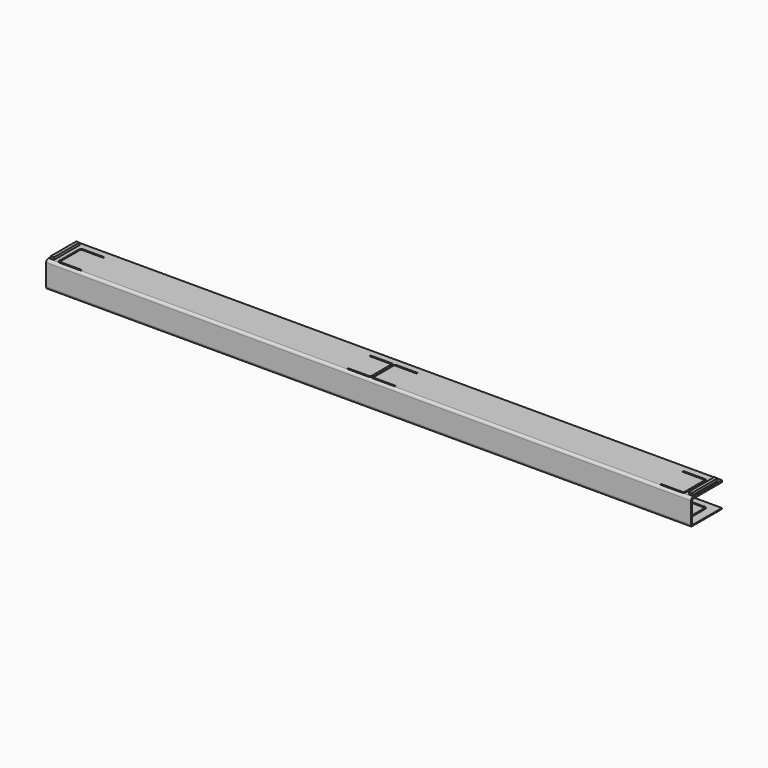
from build123d import *

# Parameters (mm, degrees)
F0_W         = 69
F0_H         = 5.7454954955
F1_DEPTH     = 2050
F2_W         = 10
F2_H         = 101.5
F3_DEPTH     = 7.5
F7_DEPTH     = 84
F10_DEPTH    = 90
F11_T1_DEPTH = 134.5
F12_T1_DEPTH = 139.5


# Not quite as in the source:
# - a fillet or chamfer that OpenCascade refuses, or shapes differently, is made with other operations: its cross-section is extruded or revolved along the edge and cut away or added


with BuildPart() as f1:
    # F0 (on Right) → F1 (new body)
    with BuildSketch(Plane.YZ):
        with BuildLine():
            ThreePointArc((-53.5, -33.75), (-51.1568542495, -39.4068542495), (-45.5, -41.75))
            Line((-45.5, -41.75), (0, -41.75))
            Line((0, -41.75), (0, -36.0045045045))
            Line((0, -36.0045045045), (-45.5, -36.0045045045))
            ThreePointArc((-45.5, -36.0045045045), (-48.3284271247, -34.8329316293), (-49.5, -32.0045045045))
            Line((-49.5, -32.0045045045), (-49.5, 32.0045045045))
            ThreePointArc((-49.5, 32.0045045045), (-48.3284271247, 34.8329316293), (-45.5, 36.0045045045))
            Line((-45.5, 36.0045045045), (0, 36.0045045045))
            Line((0, 36.0045045045), (0, 41.75))
            Line((0, 41.75), (-45.5, 41.75))
            ThreePointArc((-45.5, 41.75), (-51.1568542495, 39.4068542495), (-53.5, 33.75))
            Line((-53.5, 33.75), (-53.5, -33.75))
        make_face()
        with Locations((34.5, 38.8772522523)):
            Rectangle(F0_W, F0_H)
        with Locations((34.5, -38.8772522523)):
            Rectangle(F0_W, F0_H)
    extrude(amount=-F1_DEPTH)

    # F2 (on face) → F3 (join)
    with BuildSketch(Plane.XY.offset(41.75)):
        with Locations((-2039, 8.25)):
            Rectangle(F2_W, F2_H)
    extrude(amount=F3_DEPTH)

    # F5: F1 across plane


with BuildPart() as f1_1:
    add(f1.part)
    add(f1.part.mirror(Plane.YZ.offset(-1025)))

    # F6 (on face) → F7 (cut)
    with BuildSketch(Plane.XY.offset(41.75)):
        with BuildLine():
            Line((-2021, 39.5), (-2021, 0))
            Line((-2021, 0), (-2021, -37.5))
            ThreePointArc((-2021, -37.5), (-2018.6568542495, -43.1568542495), (-2013, -45.5))
            Line((-2013, -45.5), (-1945.5, -45.5))
            Line((-1945.5, -45.5), (-1945.5, -41.25))
            Line((-1945.5, -41.25), (-2004.9698543549, -41.25))
            Line((-2004.9698543549, -41.25), (-2012.75, -41.25))
            ThreePointArc((-2012.75, -41.25), (-2015.5784271247, -40.0784271247), (-2016.75, -37.25))
            Line((-2016.75, -37.25), (-2016.75, 0))
            Line((-2016.75, 0), (-2016.75, 39.25))
            ThreePointArc((-2016.75, 39.25), (-2015.5784271247, 42.0784271247), (-2012.75, 43.25))
            Line((-2012.75, 43.25), (-1945.5, 43.25))
            Line((-1945.5, 43.25), (-1945.5, 47.5))
            Line((-1945.5, 47.5), (-2013, 47.5))
            ThreePointArc((-2013, 47.5), (-2018.6568542495, 45.1568542495), (-2021, 39.5))
        make_face()
    extrude(amount=-F7_DEPTH, mode=Mode.SUBTRACT)

    # F8: F1 across plane


with BuildPart() as f1_2:
    add(f1_1.part)
    add(f1_1.part.mirror(Plane.YZ.offset(-1025)), mode=Mode.INTERSECT)

    # F9 (on face) → F10 (cut)
    with BuildSketch(Plane.XY.offset(41.75)):
        with BuildLine():
            ThreePointArc((-1024.0666470126, -40.75), (-1021.1231056256, -43.8556546004), (-1017, -45))
            Line((-1017, -45), (-950, -45))
            Line((-950, -45), (-950, -40.75))
            Line((-950, -40.75), (-1016.75, -40.75))
            ThreePointArc((-1016.75, -40.75), (-1019.5784271247, -39.5784271247), (-1020.75, -36.75))
            Line((-1020.75, -36.75), (-1020.75, 1.25))
            Line((-1020.75, 1.25), (-1020.75, 39.25))
            ThreePointArc((-1020.75, 39.25), (-1019.5784271247, 42.0784271247), (-1016.75, 43.25))
            Line((-1016.75, 43.25), (-950, 43.25))
            Line((-950, 43.25), (-950, 47.5))
            Line((-950, 47.5), (-1017, 47.5))
            ThreePointArc((-1017, 47.5), (-1021.1231056256, 46.3556546004), (-1024.0666470126, 43.25))
            Line((-1024.0666470126, 43.25), (-1025.9333529874, 43.25))
            ThreePointArc((-1025.9333529874, 43.25), (-1028.8768943744, 46.3556546004), (-1033, 47.5))
            Line((-1033, 47.5), (-1100, 47.5))
            Line((-1100, 47.5), (-1100, 43.25))
            Line((-1100, 43.25), (-1033.25, 43.25))
            ThreePointArc((-1033.25, 43.25), (-1030.4215728753, 42.0784271247), (-1029.25, 39.25))
            Line((-1029.25, 39.25), (-1029.25, 1.25))
            Line((-1029.25, 1.25), (-1029.25, -36.75))
            ThreePointArc((-1029.25, -36.75), (-1030.4215728753, -39.5784271247), (-1033.25, -40.75))
            Line((-1033.25, -40.75), (-1100, -40.75))
            Line((-1100, -40.75), (-1100, -45))
            Line((-1100, -45), (-1033, -45))
            ThreePointArc((-1033, -45), (-1028.8768943744, -43.8556546004), (-1025.9333529874, -40.75))
            Line((-1025.9333529874, -40.75), (-1024.0666470126, -40.75))
        make_face()
    extrude(amount=-F10_DEPTH, mode=Mode.SUBTRACT)

    # F11: fillet of radius 4 on 1 edges, made by hand

    # F11_s2 → F11_t1 (cut)
    with BuildSketch(Plane.XZ.offset(-79)):
        with BuildLine():
            ThreePointArc((-2046, -41.75), (-2048.8284271247, -40.5784271247), (-2050, -37.75))
            Line((-2050, -37.75), (-2050, -41.75))
            Line((-2050, -41.75), (-2046, -41.75))
        make_face()
    extrude(amount=F11_T1_DEPTH, mode=Mode.SUBTRACT)

    # F12: fillet of radius 5 on 1 edges, made by hand

    # F12_s2 → F12_t1 (cut)
    with BuildSketch(Plane.XZ.offset(-81.5)):
        with BuildLine():
            ThreePointArc((0, -36.75), (-1.4644660941, -40.2855339059), (-5, -41.75))
            Line((-5, -41.75), (0, -41.75))
            Line((0, -41.75), (0, -36.75))
        make_face()
    extrude(amount=F12_T1_DEPTH, mode=Mode.SUBTRACT)


solid = f1_2.part
